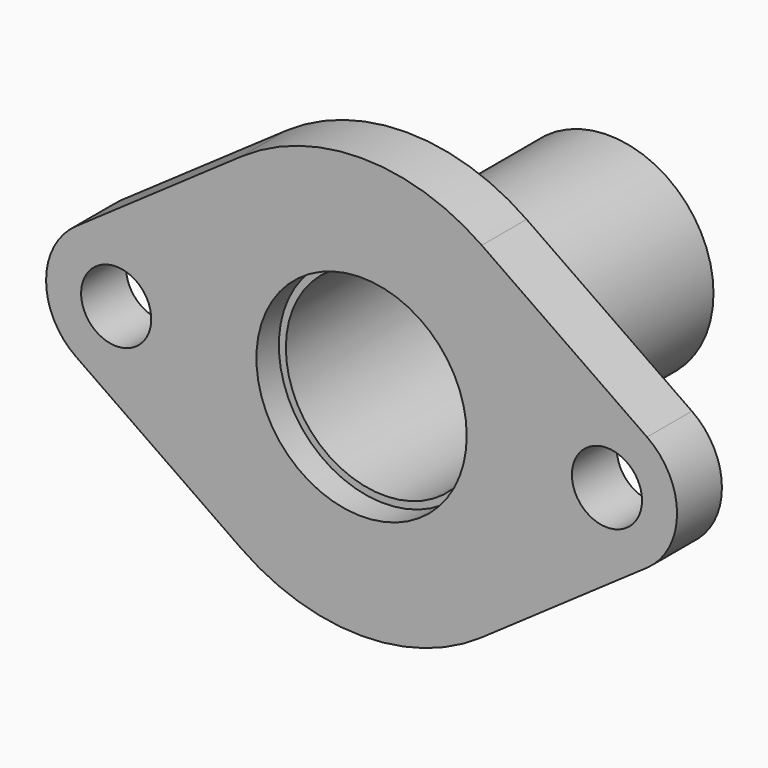
from build123d import *

# Parameters (mm, degrees)
F0_R     = 3.175
F0_R_2   = 9.525
F1_DEPTH = 2.54
F2_DEPTH = 25.4
F3_D     = 17.78


with BuildPart() as f1:
    # F0 (on Front) → F1 (new body, symmetric)
    with BuildSketch(Plane.XZ):
        with BuildLine():
            Line((-25.8535714286, -5.2111389722), (-10.8857142857, -15.6334169166))
            ThreePointArc((-10.8857142857, -15.6334169166), (0, -19.05), (10.8857142857, -15.6334169166))
            Line((10.8857142857, -15.6334169166), (25.8535714286, -5.2111389722))
            ThreePointArc((25.8535714286, -5.2111389722), (28.575, 0), (25.8535714286, 5.2111389722))
            Line((25.8535714286, 5.2111389722), (10.8857142857, 15.6334169166))
            ThreePointArc((10.8857142857, 15.6334169166), (0, 19.05), (-10.8857142857, 15.6334169166))
            Line((-10.8857142857, 15.6334169166), (-25.8535714286, 5.2111389722))
            ThreePointArc((-25.8535714286, 5.2111389722), (-28.575, 0), (-25.8535714286, -5.2111389722))
        make_face()
        with Locations((-22.225, 0)):
            Circle(F0_R, mode=Mode.SUBTRACT)
        Circle(F0_R_2, mode=Mode.SUBTRACT)
        with Locations((22.225, 0)):
            Circle(F0_R, mode=Mode.SUBTRACT)
    extrude(amount=F1_DEPTH, both=True)

    # F0 (on Front) → F2 (join)
    with BuildSketch(Plane.XZ):
        Circle(F0_R_2)
    extrude(amount=-F2_DEPTH)

    # F3 (through all)
    with Locations(Plane.XZ):
        with Locations((0, 0)):
            Hole(F3_D / 2)


solid = f1.part
